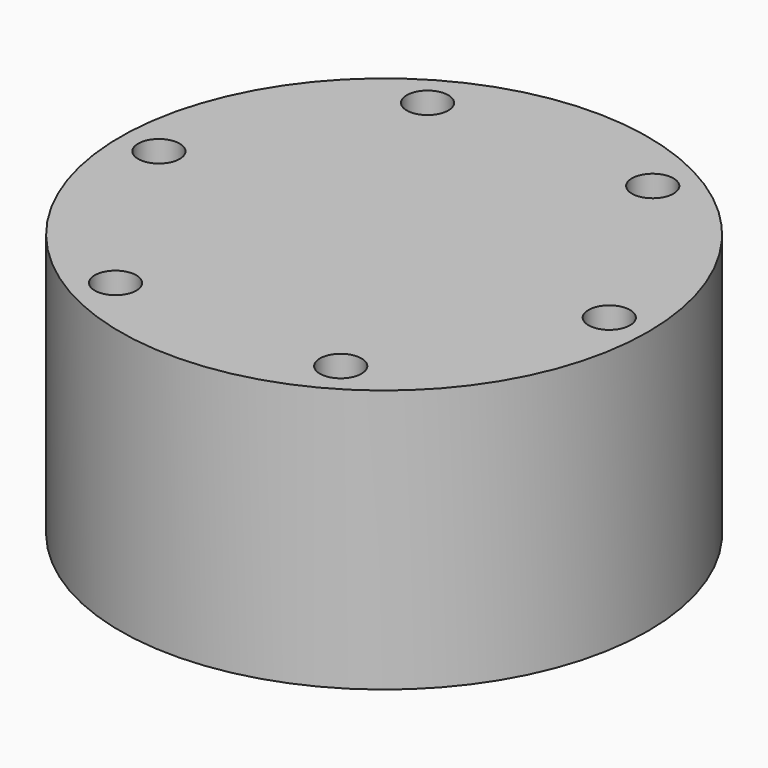
from build123d import *

# Parameters (mm, degrees)
F0_R            = 76.2
F1_DEPTH        = 76
F2_R            = 44.704
F3_DEPTH        = 50
F4_R            = 6
F5_DEPTH        = 76
F5_COPIES_COUNT = 6


# Not quite as in the source:
# - a pattern or mirror of a feature is missing from the dataset's text; its kind, count and spacing are read off the source's solid


with BuildPart() as f1:
    # F0 (on Top) → F1 (new body)
    with BuildSketch(Plane.XY):
        Circle(F0_R)
    extrude(amount=F1_DEPTH)

    # F2 (on face) → F3 (cut)
    with BuildSketch(Plane(origin=(0, 0, 0), x_dir=(1, 0, 0), z_dir=(0, 0, -1))):
        Circle(F2_R)
    extrude(amount=-F3_DEPTH, mode=Mode.SUBTRACT)

    # F4 (on face) → F5 (cut)
    with BuildSketch(Plane.XY.offset(76)):
        with Locations((-65, 0)):
            Circle(F4_R)
    f5 = extrude(amount=-F5_DEPTH, mode=Mode.SUBTRACT)

    # F5_copies: F5 ×6 about axis
    f5_copies_axis = Axis((0, 0, 0), (0, 0, 1))
    for i in range(1, F5_COPIES_COUNT):
        add(f5.rotate(f5_copies_axis, i * 360 / F5_COPIES_COUNT), mode=Mode.SUBTRACT)


solid = f1.part
